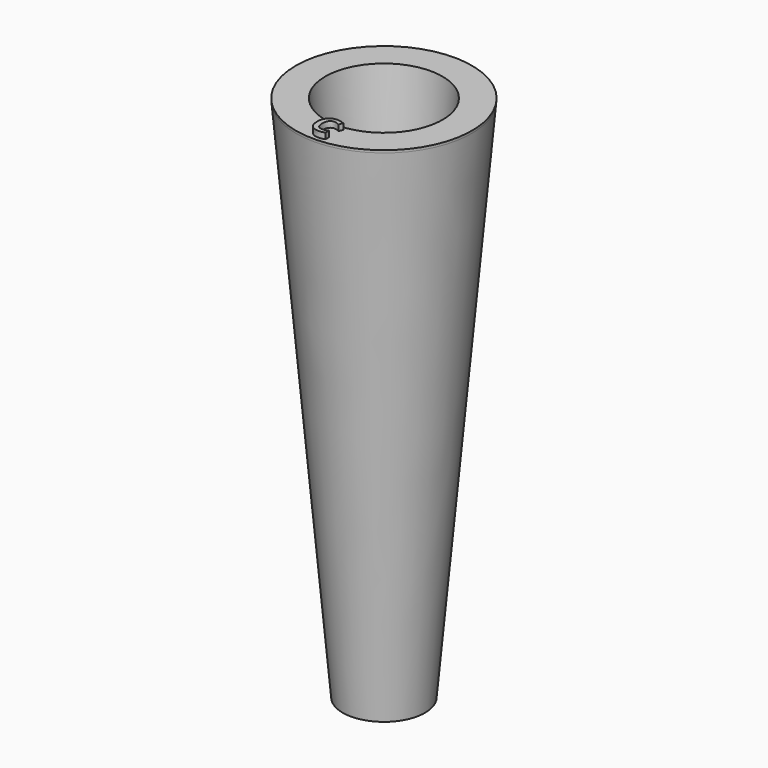
from build123d import *

# Parameters (mm, degrees)
F2_TEXT_SIZE = 5.5555555556
F3_DEPTH     = 1


# Not quite as in the source:
# - Text() gives the source's letters only with a copy of the font that has no kerning and outlines rounded to 1/6400 em; it was checked with that copy


with BuildPart() as f1:
    # F0 (on Front) → F1 (revolve)
    with BuildSketch(Plane.XZ):
        Polygon((-2, -44.6234311393), (-10, 45.3765688607), (-15.0197142214, 45.3765688607), (-14.9803632035, 44.9338699093), (-7.0197142214, -44.6234311393), align=None)
    revolve(axis=Axis((0, 0, 0.3765688607), (0, 0, -1)))

    # F2 (on face) → F3 (join)
    with BuildSketch(Plane.XY.offset(45.3765688607)):
        with Locations((-1.8524305556, -14.2680348922)):
            Text('C', F2_TEXT_SIZE, font='Open Sans', font_style=FontStyle.BOLD, text_align=(TextAlign.LEFT, TextAlign.BOTTOM))
    extrude(amount=F3_DEPTH)


solid = f1.part
